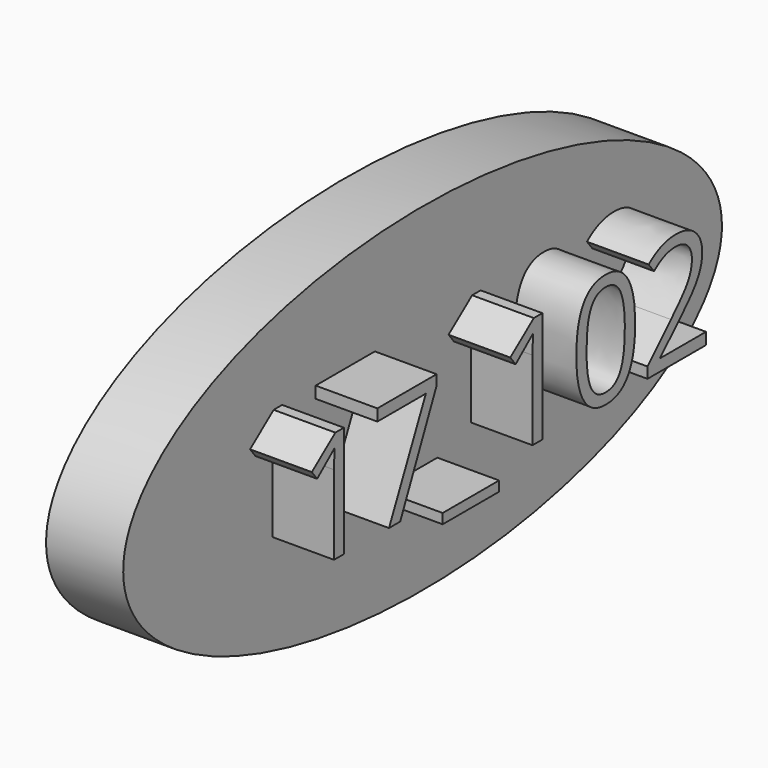
from build123d import *

# Parameters (mm, degrees)
F1_DEPTH     = 25.4
F2_TEXT_SIZE = 51.3264391985
F3_DEPTH     = 20.32


# Not quite as in the source:
# - Text() gives the source's letters only with a copy of the font that has no kerning and outlines rounded to 1/6400 em; it was checked with that copy


with BuildPart() as f1:
    # F0 (on Right) → F1 (new body)
    with BuildSketch(Plane.YZ):
        with BuildLine():
            add(Edge.make_bspline(
                [(123.2200860977, 0), (123.2200860977, 96.4108250514), (-61.6100430489, 48.2054125257), (-246.4401721954, 0), (-61.6100430489, -48.2054125257), (123.2200860977, -96.4108250514), (123.2200860977, 0)],
                knots=[0, 0, 0, 2.0943951024, 2.0943951024, 4.1887902048, 4.1887902048, 6.2831853072, 6.2831853072, 6.2831853072], degree=2, weights=[1, 0.5, 1, 0.5, 1, 0.5, 1]))
        make_face()
    extrude(amount=F1_DEPTH)

    # F2 (on face) → F3 (join)
    with BuildSketch(Plane.YZ.offset(25.4)):
        with Locations((-75.7108181715, -15.0591060519)):
            Text('17_102', F2_TEXT_SIZE, font='Open Sans', text_align=(TextAlign.LEFT, TextAlign.BOTTOM))
    extrude(amount=F3_DEPTH)


solid = f1.part
